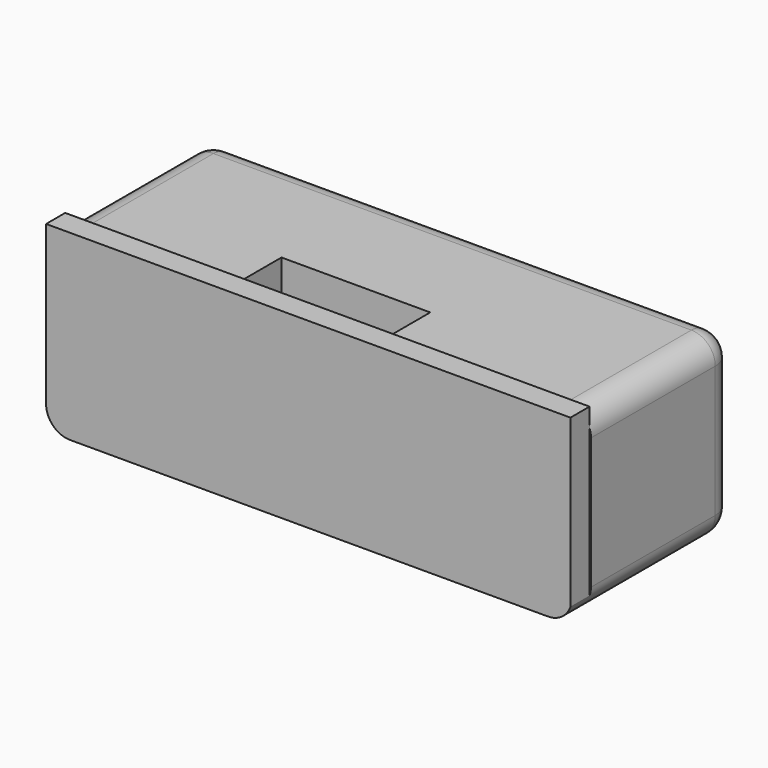
from build123d import *

# Parameters (mm, degrees)
F0_W         = 19.05
F0_H         = 19.05
F1_DEPTH     = 55.88
F2_W         = 47.625
F2_H         = 9.525
F3_DEPTH     = 25.4
F4_W         = 55.7279027998
F4_H         = 19.3847697228
F5_DEPTH     = 2.54
F6_T1_DEPTH  = 50.8
F6_T3_DEPTH  = 13.97
F6_T5_DEPTH  = 47.625
F6_T7_DEPTH  = 9.525
F6_T9_DEPTH  = 16.51
F6_T11_DEPTH = 25.4
F6_T13_DEPTH = 22.86
F6_S17_W     = 2.5908
F6_S17_H     = 2.5908
F6_T18_DEPTH = 2.5908
F6_S23_W     = 2.5908
F6_S23_H     = 2.5908
F6_T24_DEPTH = 2.5908
F6_S29_W     = 2.5908
F6_S29_H     = 2.5908
F6_T30_DEPTH = 2.5908
F6_S35_W     = 2.5908
F6_S35_H     = 2.5908
F6_T36_DEPTH = 2.5908
F6_T43_DEPTH = 53.975
F6_T48_DEPTH = 15.875
F6_T56_DEPTH = 53.975
F6_T61_DEPTH = 15.875
F6_T69_DEPTH = 15.875
F6_T74_DEPTH = 53.975
F6_T82_DEPTH = 53.975
F6_T87_DEPTH = 15.875
F7_W         = 15.8100910485
F7_H         = 5.4600955918
F8_DEPTH     = 12.7


# Not quite as in the source:
# - a fillet or chamfer that OpenCascade refuses, or shapes differently, is made with other operations: its cross-section is extruded or revolved along the edge and cut away or added


with BuildPart() as f1:
    # F0 (on Right) → F1 (new body)
    with BuildSketch(Plane.YZ):
        with Locations((9.525, 9.525)):
            Rectangle(F0_W, F0_H)
    extrude(amount=F1_DEPTH)

    # F2 (on face) → F3 (cut)
    with BuildSketch(Plane.XZ):
        with Locations((28.2575, 9.2075)):
            Rectangle(F2_W, F2_H)
    extrude(amount=-F3_DEPTH, mode=Mode.SUBTRACT)

    # F4 (on Front) → F5 (join)
    with BuildSketch(Plane.XZ):
        with Locations((27.8639513999, 9.6923848614)):
            Rectangle(F4_W, F4_H)
    extrude(amount=F5_DEPTH)

    # F6: fillet of radius 2.54 on 12 edges, made by hand

    # F6_s2 → F6_t1 (cut)
    with BuildSketch(Plane.YZ.offset(2.54)):
        with BuildLine():
            ThreePointArc((19.05, 2.54), (18.3060512242, 0.7439487758), (16.51, 0))
            Line((16.51, 0), (19.05, 0))
            Line((19.05, 0), (19.05, 2.54))
        make_face()
        with BuildLine():
            ThreePointArc((16.51, 19.05), (18.3060512242, 18.3060512242), (19.05, 16.51))
            Line((19.05, 16.51), (19.05, 19.05))
            Line((19.05, 19.05), (16.51, 19.05))
        make_face()
    extrude(amount=F6_T1_DEPTH, mode=Mode.SUBTRACT)

    # F6_s4 → F6_t3 (cut)
    with BuildSketch(Plane.XY.offset(2.54)):
        with BuildLine():
            ThreePointArc((0, 16.51), (0.7439487758, 18.3060512242), (2.54, 19.05))
            Line((2.54, 19.05), (0, 19.05))
            Line((0, 19.05), (0, 16.51))
        make_face()
        with BuildLine():
            ThreePointArc((53.34, 19.05), (55.1360512242, 18.3060512242), (55.88, 16.51))
            Line((55.88, 16.51), (55.88, 19.05))
            Line((55.88, 19.05), (53.34, 19.05))
        make_face()
    extrude(amount=F6_T3_DEPTH, mode=Mode.SUBTRACT)

    # F6_s6 → F6_t5 (cut)
    with BuildSketch(Plane.YZ.offset(4.445)):
        with BuildLine():
            ThreePointArc((19.05, 16.51), (18.3060512242, 14.7139487758), (16.51, 13.97))
            Line((16.51, 13.97), (19.05, 13.97))
            Line((19.05, 13.97), (19.05, 16.51))
        make_face()
        with BuildLine():
            ThreePointArc((19.05, 1.905), (18.3060512242, 3.7010512242), (16.51, 4.445))
            Line((16.51, 4.445), (19.05, 4.445))
            Line((19.05, 4.445), (19.05, 1.905))
        make_face()
    extrude(amount=F6_T5_DEPTH, mode=Mode.SUBTRACT)

    # F6_s8 → F6_t7 (cut)
    with BuildSketch(Plane.XY.offset(4.445)):
        with BuildLine():
            ThreePointArc((1.905, 19.05), (3.7010512242, 18.3060512242), (4.445, 16.51))
            Line((4.445, 16.51), (4.445, 19.05))
            Line((4.445, 19.05), (1.905, 19.05))
        make_face()
        with BuildLine():
            ThreePointArc((54.61, 19.05), (52.8139487758, 18.3060512242), (52.07, 16.51))
            Line((52.07, 16.51), (52.07, 19.05))
            Line((52.07, 19.05), (54.61, 19.05))
        make_face()
    extrude(amount=F6_T7_DEPTH, mode=Mode.SUBTRACT)

    # F6_s10 → F6_t9 (cut)
    with BuildSketch(Plane.XZ.offset(-16.51)):
        with BuildLine():
            ThreePointArc((2.54, 19.05), (0.7439487758, 18.3060512242), (0, 16.51))
            Line((0, 16.51), (0, 19.05))
            Line((0, 19.05), (2.54, 19.05))
        make_face()
        with BuildLine():
            ThreePointArc((53.34, 19.05), (55.1360512242, 18.3060512242), (55.88, 16.51))
            Line((55.88, 16.51), (55.88, 19.05))
            Line((55.88, 19.05), (53.34, 19.05))
        make_face()
    extrude(amount=F6_T9_DEPTH, mode=Mode.SUBTRACT)

    # F6_s12 → F6_t11 (cut)
    with BuildSketch(Plane.XZ.offset(-16.51)):
        with BuildLine():
            ThreePointArc((0, 2.54), (0.7439487758, 0.7439487758), (2.54, 0))
            Line((2.54, 0), (0, 0))
            Line((0, 0), (0, 2.54))
        make_face()
    extrude(amount=F6_T11_DEPTH, mode=Mode.SUBTRACT)

    # F6_s14 → F6_t13 (cut)
    with BuildSketch(Plane.XZ.offset(-16.51)):
        with BuildLine():
            ThreePointArc((55.88, 2.54), (55.1360512242, 0.7439487758), (53.34, 0))
            Line((53.34, 0), (55.88, 0))
            Line((55.88, 0), (55.88, 2.54))
        make_face()
    extrude(amount=F6_T13_DEPTH, mode=Mode.SUBTRACT)


with BuildPart() as f6_tool16:
    # F6_s17 → F6_t18 (new body)
    with BuildSketch(Plane.YZ.offset(2.54)):
        with Locations((17.8054, 1.2446)):
            Rectangle(F6_S17_W, F6_S17_H)
    extrude(amount=-F6_T18_DEPTH)

    # F6_s19 → F6_t20 (revolve, cut)
    with BuildSketch(Plane(origin=(2.54, 16.51, 2.54), x_dir=(0, -0.7071067812, 0.7071067812), z_dir=(0, -0.7071067812, -0.7071067812))):
        with BuildLine():
            ThreePointArc((0, -2.54), (2.54, 0), (0, 2.54))
            Line((0, 2.54), (0, -2.54))
        make_face()
    revolve(axis=Axis((2.54, 16.51, 2.54), (-1, 0, 0)), mode=Mode.SUBTRACT)


with BuildPart() as f1_1:
    add(f1.part)

    # F6_t15: cut F6_tool16
    add(f6_tool16.part, mode=Mode.SUBTRACT)


with BuildPart() as f6_tool22:
    # F6_s23 → F6_t24 (new body)
    with BuildSketch(Plane.YZ.offset(53.34)):
        with Locations((17.8054, 1.2446)):
            Rectangle(F6_S23_W, F6_S23_H)
    extrude(amount=F6_T24_DEPTH)

    # F6_s25 → F6_t26 (revolve, cut)
    with BuildSketch(Plane(origin=(53.34, 16.51, 2.54), x_dir=(0, -0.7071067812, 0.7071067812), z_dir=(0, 0.7071067812, 0.7071067812))):
        with BuildLine():
            ThreePointArc((0, -2.54), (2.54, 0), (0, 2.54))
            Line((0, 2.54), (0, -2.54))
        make_face()
    revolve(axis=Axis((53.34, 16.51, 2.54), (1, 0, 0)), mode=Mode.SUBTRACT)


with BuildPart() as f1_2:
    add(f1_1.part)

    # F6_t21: cut F6_tool22
    add(f6_tool22.part, mode=Mode.SUBTRACT)


with BuildPart() as f6_tool28:
    # F6_s29 → F6_t30 (new body)
    with BuildSketch(Plane.XY.offset(16.51)):
        with Locations((1.2446, 17.8054)):
            Rectangle(F6_S29_W, F6_S29_H)
    extrude(amount=F6_T30_DEPTH)

    # F6_s31 → F6_t32 (revolve, cut)
    with BuildSketch(Plane(origin=(2.54, 16.51, 16.51), x_dir=(0.7071067812, -0.7071067812, 0), z_dir=(-0.7071067812, -0.7071067812, 0))):
        with BuildLine():
            ThreePointArc((0, -2.54), (2.54, 0), (0, 2.54))
            Line((0, 2.54), (0, -2.54))
        make_face()
    revolve(axis=Axis((2.54, 16.51, 16.51), (0, 0, 1)), mode=Mode.SUBTRACT)


with BuildPart() as f1_3:
    add(f1_2.part)

    # F6_t27: cut F6_tool28
    add(f6_tool28.part, mode=Mode.SUBTRACT)


with BuildPart() as f6_tool34:
    # F6_s35 → F6_t36 (new body)
    with BuildSketch(Plane.XY.offset(16.51)):
        with Locations((54.6354, 17.8054)):
            Rectangle(F6_S35_W, F6_S35_H)
    extrude(amount=F6_T36_DEPTH)

    # F6_s37 → F6_t38 (revolve, cut)
    with BuildSketch(Plane(origin=(53.34, 16.51, 16.51), x_dir=(-0.7071067812, -0.7071067812, 0), z_dir=(-0.7071067812, 0.7071067812, 0))):
        with BuildLine():
            ThreePointArc((0, -2.54), (2.54, 0), (0, 2.54))
            Line((0, 2.54), (0, -2.54))
        make_face()
    revolve(axis=Axis((53.34, 16.51, 16.51), (0, 0, 1)), mode=Mode.SUBTRACT)


with BuildPart() as f1_4:
    add(f1_3.part)

    # F6_t33: cut F6_tool34
    add(f6_tool34.part, mode=Mode.SUBTRACT)


with BuildPart() as f6_tool41:
    # F6_s42 → F6_t43 (new body)
    with BuildSketch(Plane.YZ.offset(58.42)):
        with BuildLine():
            ThreePointArc((19.05, 16.51), (18.3060512242, 14.7139487758), (16.51, 13.97))
            Line((16.51, 13.97), (19.05, 13.97))
            Line((19.05, 13.97), (19.05, 16.51))
        make_face()
    extrude(amount=-F6_T43_DEPTH)

    split(bisect_by=Plane.YZ.offset(52.07), keep=Keep.TOP)

    split(bisect_by=Plane.YZ.offset(55.88), keep=Keep.BOTTOM)


with BuildPart() as f6_tool46:
    # F6_s47 → F6_t48 (new body)
    with BuildSketch(Plane.XY.offset(4.445)):
        with BuildLine():
            ThreePointArc((54.61, 19.05), (52.8139487758, 18.3060512242), (52.07, 16.51))
            Line((52.07, 16.51), (52.07, 19.05))
            Line((52.07, 19.05), (54.61, 19.05))
        make_face()
    extrude(amount=F6_T48_DEPTH)

    split(bisect_by=Plane.XY.offset(19.05), keep=Keep.BOTTOM)

    split(bisect_by=Plane.XY.offset(13.97), keep=Keep.TOP)


with BuildPart() as f6_tool41_1:
    add(f6_tool41.part)

    # F6_t51: intersect F6_tool46
    add(f6_tool46.part, mode=Mode.INTERSECT)


with BuildPart() as f1_5:
    add(f1_4.part)

    # F6_t39: cut F6_tool41
    add(f6_tool41_1.part, mode=Mode.SUBTRACT)


with BuildPart() as f6_tool54:
    # F6_s55 → F6_t56 (new body)
    with BuildSketch(Plane.YZ.offset(52.07)):
        with BuildLine():
            ThreePointArc((19.05, 16.51), (18.3060512242, 14.7139487758), (16.51, 13.97))
            Line((16.51, 13.97), (19.05, 13.97))
            Line((19.05, 13.97), (19.05, 16.51))
        make_face()
    extrude(amount=-F6_T56_DEPTH)

    split(bisect_by=Plane.YZ, keep=Keep.TOP)

    split(bisect_by=Plane.YZ.offset(4.445), keep=Keep.BOTTOM)


with BuildPart() as f6_tool59:
    # F6_s60 → F6_t61 (new body)
    with BuildSketch(Plane.XY.offset(20.32)):
        with BuildLine():
            ThreePointArc((1.905, 19.05), (3.7010512242, 18.3060512242), (4.445, 16.51))
            Line((4.445, 16.51), (4.445, 19.05))
            Line((4.445, 19.05), (1.905, 19.05))
        make_face()
    extrude(amount=-F6_T61_DEPTH)

    split(bisect_by=Plane.XY.offset(19.05), keep=Keep.BOTTOM)

    split(bisect_by=Plane.XY.offset(13.97), keep=Keep.TOP)


with BuildPart() as f6_tool54_1:
    add(f6_tool54.part)

    # F6_t64: intersect F6_tool59
    add(f6_tool59.part, mode=Mode.INTERSECT)


with BuildPart() as f1_6:
    add(f1_5.part)

    # F6_t52: cut F6_tool54
    add(f6_tool54_1.part, mode=Mode.SUBTRACT)


with BuildPart() as f6_tool67:
    # F6_s68 → F6_t69 (new body)
    with BuildSketch(Plane.XY.offset(13.97)):
        with BuildLine():
            ThreePointArc((1.905, 19.05), (3.7010512242, 18.3060512242), (4.445, 16.51))
            Line((4.445, 16.51), (4.445, 19.05))
            Line((4.445, 19.05), (1.905, 19.05))
        make_face()
    extrude(amount=-F6_T69_DEPTH)

    split(bisect_by=Plane.XY.offset(4.445), keep=Keep.BOTTOM)

    split(bisect_by=Plane.XY, keep=Keep.TOP)


with BuildPart() as f6_tool72:
    # F6_s73 → F6_t74 (new body)
    with BuildSketch(Plane.YZ.offset(-1.905)):
        with BuildLine():
            ThreePointArc((19.05, 1.905), (18.3060512242, 3.7010512242), (16.51, 4.445))
            Line((16.51, 4.445), (19.05, 4.445))
            Line((19.05, 4.445), (19.05, 1.905))
        make_face()
    extrude(amount=F6_T74_DEPTH)

    split(bisect_by=Plane.YZ, keep=Keep.TOP)

    split(bisect_by=Plane.YZ.offset(4.445), keep=Keep.BOTTOM)


with BuildPart() as f6_tool67_1:
    add(f6_tool67.part)

    # F6_t77: intersect F6_tool72
    add(f6_tool72.part, mode=Mode.INTERSECT)


with BuildPart() as f1_7:
    add(f1_6.part)

    # F6_t65: cut F6_tool67
    add(f6_tool67_1.part, mode=Mode.SUBTRACT)


with BuildPart() as f6_tool80:
    # F6_s81 → F6_t82 (new body)
    with BuildSketch(Plane.YZ.offset(4.445)):
        with BuildLine():
            ThreePointArc((19.05, 1.905), (18.3060512242, 3.7010512242), (16.51, 4.445))
            Line((16.51, 4.445), (19.05, 4.445))
            Line((19.05, 4.445), (19.05, 1.905))
        make_face()
    extrude(amount=F6_T82_DEPTH)

    split(bisect_by=Plane.YZ.offset(52.07), keep=Keep.TOP)

    split(bisect_by=Plane.YZ.offset(55.88), keep=Keep.BOTTOM)


with BuildPart() as f6_tool85:
    # F6_s86 → F6_t87 (new body)
    with BuildSketch(Plane.XY.offset(-1.905)):
        with BuildLine():
            ThreePointArc((54.61, 19.05), (52.8139487758, 18.3060512242), (52.07, 16.51))
            Line((52.07, 16.51), (52.07, 19.05))
            Line((52.07, 19.05), (54.61, 19.05))
        make_face()
    extrude(amount=F6_T87_DEPTH)

    split(bisect_by=Plane.XY.offset(4.445), keep=Keep.BOTTOM)

    split(bisect_by=Plane.XY, keep=Keep.TOP)


with BuildPart() as f6_tool80_1:
    add(f6_tool80.part)

    # F6_t90: intersect F6_tool85
    add(f6_tool85.part, mode=Mode.INTERSECT)


with BuildPart() as f1_8:
    add(f1_7.part)

    # F6_t78: cut F6_tool80
    add(f6_tool80_1.part, mode=Mode.SUBTRACT)

    # F7 (on face) → F8 (cut)
    with BuildSketch(Plane.XY.offset(19.05)):
        with Locations((26.5251491219, 2.7300477959)):
            Rectangle(F7_W, F7_H)
    extrude(amount=-F8_DEPTH, mode=Mode.SUBTRACT)


solid = f1_8.part
